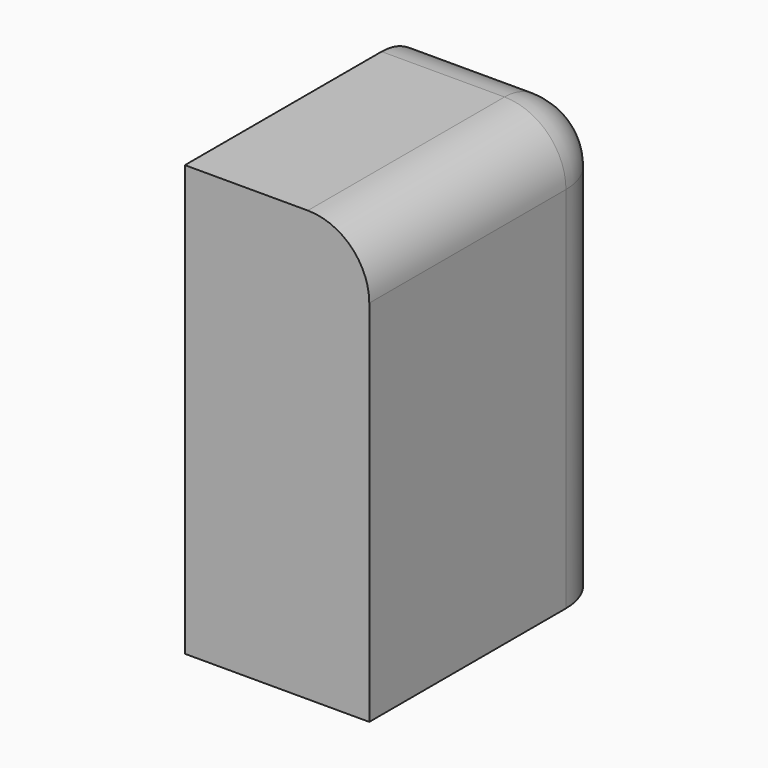
from build123d import *

# Parameters (mm, degrees)
F0_W     = 30
F0_H     = 50
F1_DEPTH = 70
F3_R     = 10


# Not quite as in the source:
# - a feature of the source that left no trace in its solid (it failed there, or was rolled back) is left out


with BuildPart() as f1:
    # F0 (on Top) → F1 (new body)
    with BuildSketch(Plane.XY):
        with Locations((-0.0802149171, 25)):
            Rectangle(F0_W, F0_H)
    extrude(amount=F1_DEPTH)


with BuildPart() as f1_1:
    # F2: moved
    add(f1.part.moved(Location((30, 50, 70))))

    # F3
    f3_edges = [f1_1.edges().sort_by_distance(p)[0] for p in [
        (44.919785, 75, 140),
        (29.919785, 100, 140),
        (44.919785, 100, 105),
    ]]
    fillet(f3_edges, radius=F3_R)


solid = f1_1.part
